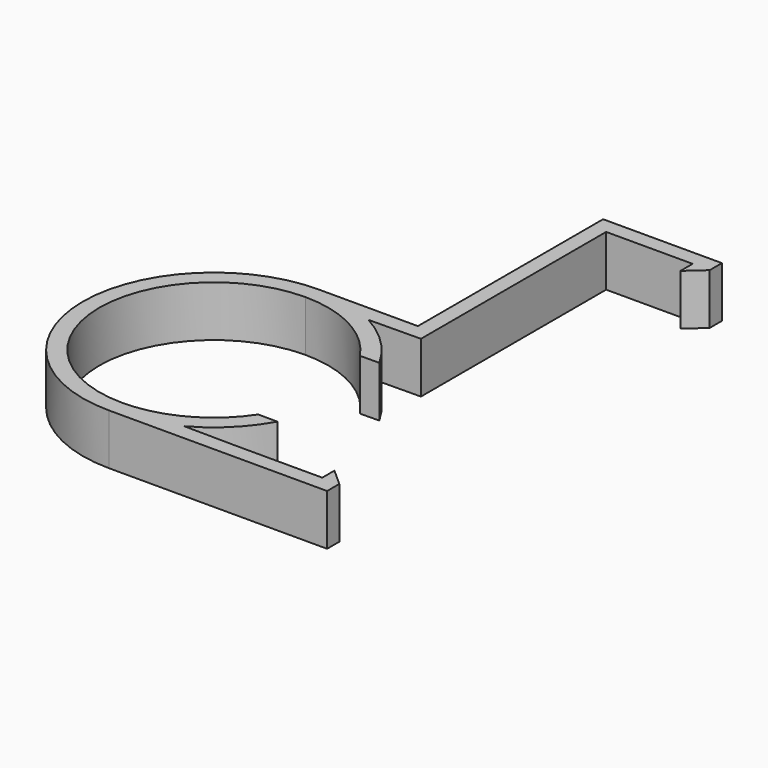
from build123d import *

# Parameters (mm, degrees)
F1_DEPTH = 10


# Not quite as in the source:
# - a feature names something its author has since deleted; it is built from what else it names


with BuildPart() as f1:
    # F0 (on Top) → F1 (new body)
    with BuildSketch(Plane.XY):
        with BuildLine():
            Line((-18.9642689968, 23.316359701), (-38.4642689968, 23.316359701))
            ThreePointArc((-38.4642689968, 23.316359701), (-56.6722686123, 15.7743593166), (-64.2142689968, -2.433640299))
            ThreePointArc((-64.2142689968, -2.433640299), (-56.6722686123, -20.6416399145), (-38.4642689968, -28.183640299))
            Line((-38.4642689968, -28.183640299), (4.3898329695, -28.183640299))
            Line((4.3898329695, -28.183640299), (4.3898329695, -25.183640299))
            Line((4.3898329695, -25.183640299), (1.0357310032, -22.183640299))
            Line((1.0357310032, -22.183640299), (1.0357310032, -25.183640299))
            Line((1.0357310032, -25.183640299), (-15.9642689968, -25.183640299))
            Line((-15.9642689968, -25.183640299), (-26.1900364695, -25.0700206604))
            Line((-26.1900364695, -25.0700206604), (-38.4642689968, -24.933640299))
            ThreePointArc((-38.4642689968, -24.933640299), (-54.3741715735, -18.3435428757), (-60.9642689968, -2.433640299))
            ThreePointArc((-60.9642689968, -2.433640299), (-54.3741715735, 13.4762622777), (-38.4642689968, 20.066359701))
            ThreePointArc((-38.4642689968, 20.066359701), (-27.8473278519, 17.4039644135), (-19.7429639579, 10.0468539878))
            Line((-19.7429639579, 10.0468539878), (-15.9642689968, 10.0888394874))
            ThreePointArc((-15.9642689968, 10.0888394874), (-20.3566861052, 15.8742252736), (-26.1900364695, 20.2027400624))
            Line((-26.1900364695, 20.2027400624), (-15.9642689968, 20.316359701))
            Line((-15.9642689968, 20.316359701), (-15.9642689968, 65.816359701))
            Line((-15.9642689968, 65.816359701), (1.0357310032, 65.816359701))
            Line((1.0357310032, 65.816359701), (1.0357310032, 62.816359701))
            Line((1.0357310032, 62.816359701), (4.3898329695, 65.816359701))
            Line((4.3898329695, 65.816359701), (4.3898329695, 68.816359701))
            Line((4.3898329695, 68.816359701), (-15.9642689968, 68.816359701))
            Line((-15.9642689968, 68.816359701), (-18.9642689968, 68.816359701))
            Line((-18.9642689968, 68.816359701), (-18.9642689968, 23.316359701))
        make_face()
        with BuildLine():
            Line((-38.4642689968, -24.933640299), (-26.1900364695, -25.0700206604))
            ThreePointArc((-26.1900364695, -25.0700206604), (-20.3566861052, -20.7415058716), (-15.9642689968, -14.9561200853))
            Line((-15.9642689968, -14.9561200853), (-19.7429639579, -14.9141345858))
            ThreePointArc((-19.7429639579, -14.9141345858), (-27.8473278519, -22.2712450114), (-38.4642689968, -24.933640299))
        make_face()
    extrude(amount=F1_DEPTH)


solid = f1.part
